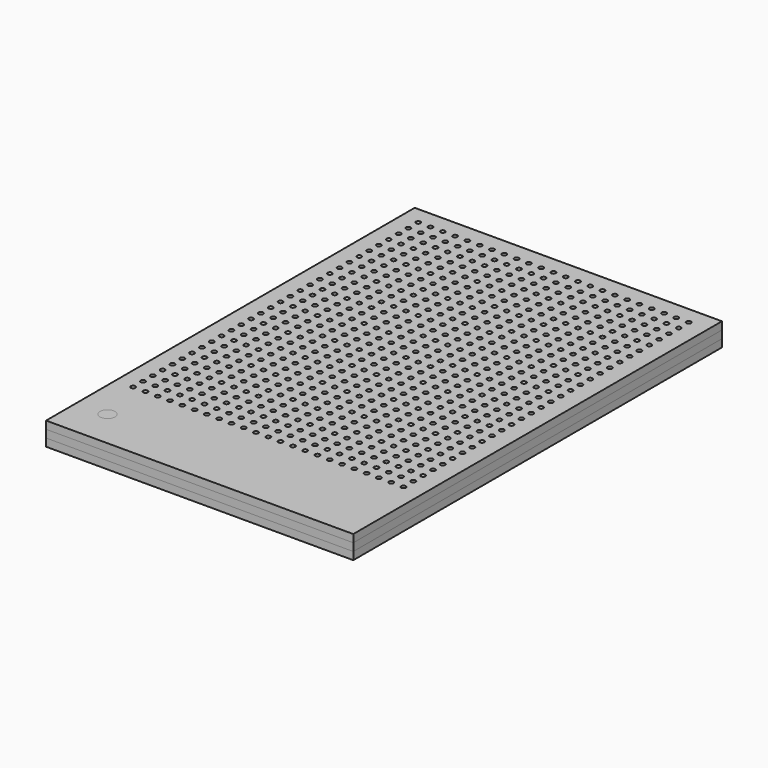
from build123d import *

# Parameters (mm, degrees)
F0_W      = 200
F0_H      = 300
F1_DEPTH  = 5
F2_R      = 1.5
F3_DEPTH  = 5.001
F4_W      = 200
F4_H      = 300
F5_DEPTH  = 5
F6_W      = 3
F6_H      = 235
F7_DEPTH  = 4
F8_R      = 4.875
F9_DEPTH  = 5
F10_DEPTH = 5
F11_R     = 4.875
F12_DEPTH = 0.5


with BuildPart() as f1:
    # F0 (on Top) → F1 (new body)
    with BuildSketch(Plane.XY):
        with Locations((100, 150)):
            Rectangle(F0_W, F0_H)
    extrude(amount=F1_DEPTH)

    # F2 (on face) → F3 (cut, through all)
    with BuildSketch(Plane.XY.offset(5)):
        with Locations((11.5, 288.5)):
            Circle(F2_R)
        with Locations((11.5, 280.5)):
            Circle(F2_R)
        with Locations((11.5, 272.5)):
            Circle(F2_R)
        with Locations((11.5, 264.5)):
            Circle(F2_R)
        with Locations((11.5, 256.5)):
            Circle(F2_R)
        with Locations((11.5, 248.5)):
            Circle(F2_R)
        with Locations((11.5, 240.5)):
            Circle(F2_R)
        with Locations((11.5, 232.5)):
            Circle(F2_R)
        with Locations((11.5, 224.5)):
            Circle(F2_R)
        with Locations((11.5, 216.5)):
            Circle(F2_R)
        with Locations((11.5, 208.5)):
            Circle(F2_R)
        with Locations((11.5, 200.5)):
            Circle(F2_R)
        with Locations((11.5, 192.5)):
            Circle(F2_R)
        with Locations((11.5, 184.5)):
            Circle(F2_R)
        with Locations((11.5, 176.5)):
            Circle(F2_R)
        with Locations((11.5, 168.5)):
            Circle(F2_R)
        with Locations((11.5, 160.5)):
            Circle(F2_R)
        with Locations((11.5, 152.5)):
            Circle(F2_R)
        with Locations((11.5, 144.5)):
            Circle(F2_R)
        with Locations((11.5, 136.5)):
            Circle(F2_R)
        with Locations((11.5, 128.5)):
            Circle(F2_R)
        with Locations((11.5, 120.5)):
            Circle(F2_R)
        with Locations((11.5, 112.5)):
            Circle(F2_R)
        with Locations((11.5, 104.5)):
            Circle(F2_R)
        with Locations((19.5, 288.5)):
            Circle(F2_R)
        with Locations((19.5, 280.5)):
            Circle(F2_R)
        with Locations((19.5, 272.5)):
            Circle(F2_R)
        with Locations((19.5, 264.5)):
            Circle(F2_R)
        with Locations((19.5, 256.5)):
            Circle(F2_R)
        with Locations((19.5, 248.5)):
            Circle(F2_R)
        with Locations((19.5, 240.5)):
            Circle(F2_R)
        with Locations((19.5, 232.5)):
            Circle(F2_R)
        with Locations((19.5, 224.5)):
            Circle(F2_R)
        with Locations((19.5, 216.5)):
            Circle(F2_R)
        with Locations((19.5, 208.5)):
            Circle(F2_R)
        with Locations((19.5, 200.5)):
            Circle(F2_R)
        with Locations((19.5, 192.5)):
            Circle(F2_R)
        with Locations((19.5, 184.5)):
            Circle(F2_R)
        with Locations((19.5, 176.5)):
            Circle(F2_R)
        with Locations((19.5, 168.5)):
            Circle(F2_R)
        with Locations((19.5, 160.5)):
            Circle(F2_R)
        with Locations((19.5, 152.5)):
            Circle(F2_R)
        with Locations((19.5, 144.5)):
            Circle(F2_R)
        with Locations((19.5, 136.5)):
            Circle(F2_R)
        with Locations((19.5, 128.5)):
            Circle(F2_R)
        with Locations((19.5, 120.5)):
            Circle(F2_R)
        with Locations((19.5, 112.5)):
            Circle(F2_R)
        with Locations((19.5, 104.5)):
            Circle(F2_R)
        with Locations((27.5, 288.5)):
            Circle(F2_R)
        with Locations((27.5, 280.5)):
            Circle(F2_R)
        with Locations((27.5, 272.5)):
            Circle(F2_R)
        with Locations((27.5, 264.5)):
            Circle(F2_R)
        with Locations((27.5, 256.5)):
            Circle(F2_R)
        with Locations((27.5, 248.5)):
            Circle(F2_R)
        with Locations((27.5, 240.5)):
            Circle(F2_R)
        with Locations((27.5, 232.5)):
            Circle(F2_R)
        with Locations((27.5, 224.5)):
            Circle(F2_R)
        with Locations((27.5, 216.5)):
            Circle(F2_R)
        with Locations((27.5, 208.5)):
            Circle(F2_R)
        with Locations((27.5, 200.5)):
            Circle(F2_R)
        with Locations((27.5, 192.5)):
            Circle(F2_R)
        with Locations((27.5, 184.5)):
            Circle(F2_R)
        with Locations((27.5, 176.5)):
            Circle(F2_R)
        with Locations((27.5, 168.5)):
            Circle(F2_R)
        with Locations((27.5, 160.5)):
            Circle(F2_R)
        with Locations((27.5, 152.5)):
            Circle(F2_R)
        with Locations((27.5, 144.5)):
            Circle(F2_R)
        with Locations((27.5, 136.5)):
            Circle(F2_R)
        with Locations((27.5, 128.5)):
            Circle(F2_R)
        with Locations((27.5, 120.5)):
            Circle(F2_R)
        with Locations((27.5, 112.5)):
            Circle(F2_R)
        with Locations((27.5, 104.5)):
            Circle(F2_R)
        with Locations((35.5, 288.5)):
            Circle(F2_R)
        with Locations((35.5, 280.5)):
            Circle(F2_R)
        with Locations((35.5, 272.5)):
            Circle(F2_R)
        with Locations((35.5, 264.5)):
            Circle(F2_R)
        with Locations((35.5, 256.5)):
            Circle(F2_R)
        with Locations((35.5, 248.5)):
            Circle(F2_R)
        with Locations((35.5, 240.5)):
            Circle(F2_R)
        with Locations((35.5, 232.5)):
            Circle(F2_R)
        with Locations((35.5, 224.5)):
            Circle(F2_R)
        with Locations((35.5, 216.5)):
            Circle(F2_R)
        with Locations((35.5, 208.5)):
            Circle(F2_R)
        with Locations((35.5, 200.5)):
            Circle(F2_R)
        with Locations((35.5, 192.5)):
            Circle(F2_R)
        with Locations((35.5, 184.5)):
            Circle(F2_R)
        with Locations((35.5, 176.5)):
            Circle(F2_R)
        with Locations((35.5, 168.5)):
            Circle(F2_R)
        with Locations((35.5, 160.5)):
            Circle(F2_R)
        with Locations((35.5, 152.5)):
            Circle(F2_R)
        with Locations((35.5, 144.5)):
            Circle(F2_R)
        with Locations((35.5, 136.5)):
            Circle(F2_R)
        with Locations((35.5, 128.5)):
            Circle(F2_R)
        with Locations((35.5, 120.5)):
            Circle(F2_R)
        with Locations((35.5, 112.5)):
            Circle(F2_R)
        with Locations((35.5, 104.5)):
            Circle(F2_R)
        with Locations((43.5, 288.5)):
            Circle(F2_R)
        with Locations((43.5, 280.5)):
            Circle(F2_R)
        with Locations((43.5, 272.5)):
            Circle(F2_R)
        with Locations((43.5, 264.5)):
            Circle(F2_R)
        with Locations((43.5, 256.5)):
            Circle(F2_R)
        with Locations((43.5, 248.5)):
            Circle(F2_R)
        with Locations((43.5, 240.5)):
            Circle(F2_R)
        with Locations((43.5, 232.5)):
            Circle(F2_R)
        with Locations((43.5, 224.5)):
            Circle(F2_R)
        with Locations((43.5, 216.5)):
            Circle(F2_R)
        with Locations((43.5, 208.5)):
            Circle(F2_R)
        with Locations((43.5, 200.5)):
            Circle(F2_R)
        with Locations((43.5, 192.5)):
            Circle(F2_R)
        with Locations((43.5, 184.5)):
            Circle(F2_R)
        with Locations((43.5, 176.5)):
            Circle(F2_R)
        with Locations((43.5, 168.5)):
            Circle(F2_R)
        with Locations((43.5, 160.5)):
            Circle(F2_R)
        with Locations((43.5, 152.5)):
            Circle(F2_R)
        with Locations((43.5, 144.5)):
            Circle(F2_R)
        with Locations((43.5, 136.5)):
            Circle(F2_R)
        with Locations((43.5, 128.5)):
            Circle(F2_R)
        with Locations((43.5, 120.5)):
            Circle(F2_R)
        with Locations((43.5, 112.5)):
            Circle(F2_R)
        with Locations((43.5, 104.5)):
            Circle(F2_R)
        with Locations((51.5, 288.5)):
            Circle(F2_R)
        with Locations((51.5, 280.5)):
            Circle(F2_R)
        with Locations((51.5, 272.5)):
            Circle(F2_R)
        with Locations((51.5, 264.5)):
            Circle(F2_R)
        with Locations((51.5, 256.5)):
            Circle(F2_R)
        with Locations((51.5, 248.5)):
            Circle(F2_R)
        with Locations((51.5, 240.5)):
            Circle(F2_R)
        with Locations((51.5, 232.5)):
            Circle(F2_R)
        with Locations((51.5, 224.5)):
            Circle(F2_R)
        with Locations((51.5, 216.5)):
            Circle(F2_R)
        with Locations((51.5, 208.5)):
            Circle(F2_R)
        with Locations((51.5, 200.5)):
            Circle(F2_R)
        with Locations((51.5, 192.5)):
            Circle(F2_R)
        with Locations((51.5, 184.5)):
            Circle(F2_R)
        with Locations((51.5, 176.5)):
            Circle(F2_R)
        with Locations((51.5, 168.5)):
            Circle(F2_R)
        with Locations((51.5, 160.5)):
            Circle(F2_R)
        with Locations((51.5, 152.5)):
            Circle(F2_R)
        with Locations((51.5, 144.5)):
            Circle(F2_R)
        with Locations((51.5, 136.5)):
            Circle(F2_R)
        with Locations((51.5, 128.5)):
            Circle(F2_R)
        with Locations((51.5, 120.5)):
            Circle(F2_R)
        with Locations((51.5, 112.5)):
            Circle(F2_R)
        with Locations((51.5, 104.5)):
            Circle(F2_R)
        with Locations((59.5, 288.5)):
            Circle(F2_R)
        with Locations((59.5, 280.5)):
            Circle(F2_R)
        with Locations((59.5, 272.5)):
            Circle(F2_R)
        with Locations((59.5, 264.5)):
            Circle(F2_R)
        with Locations((59.5, 256.5)):
            Circle(F2_R)
        with Locations((59.5, 248.5)):
            Circle(F2_R)
        with Locations((59.5, 240.5)):
            Circle(F2_R)
        with Locations((59.5, 232.5)):
            Circle(F2_R)
        with Locations((59.5, 224.5)):
            Circle(F2_R)
        with Locations((59.5, 216.5)):
            Circle(F2_R)
        with Locations((59.5, 208.5)):
            Circle(F2_R)
        with Locations((59.5, 200.5)):
            Circle(F2_R)
        with Locations((59.5, 192.5)):
            Circle(F2_R)
        with Locations((59.5, 184.5)):
            Circle(F2_R)
        with Locations((59.5, 176.5)):
            Circle(F2_R)
        with Locations((59.5, 168.5)):
            Circle(F2_R)
        with Locations((59.5, 160.5)):
            Circle(F2_R)
        with Locations((59.5, 152.5)):
            Circle(F2_R)
        with Locations((59.5, 144.5)):
            Circle(F2_R)
        with Locations((59.5, 136.5)):
            Circle(F2_R)
        with Locations((59.5, 128.5)):
            Circle(F2_R)
        with Locations((59.5, 120.5)):
            Circle(F2_R)
        with Locations((59.5, 112.5)):
            Circle(F2_R)
        with Locations((59.5, 104.5)):
            Circle(F2_R)
        with Locations((67.5, 288.5)):
            Circle(F2_R)
        with Locations((67.5, 280.5)):
            Circle(F2_R)
        with Locations((67.5, 272.5)):
            Circle(F2_R)
        with Locations((67.5, 264.5)):
            Circle(F2_R)
        with Locations((67.5, 256.5)):
            Circle(F2_R)
        with Locations((67.5, 248.5)):
            Circle(F2_R)
        with Locations((67.5, 240.5)):
            Circle(F2_R)
        with Locations((67.5, 232.5)):
            Circle(F2_R)
        with Locations((67.5, 224.5)):
            Circle(F2_R)
        with Locations((67.5, 216.5)):
            Circle(F2_R)
        with Locations((67.5, 208.5)):
            Circle(F2_R)
        with Locations((67.5, 200.5)):
            Circle(F2_R)
        with Locations((67.5, 192.5)):
            Circle(F2_R)
        with Locations((67.5, 184.5)):
            Circle(F2_R)
        with Locations((67.5, 176.5)):
            Circle(F2_R)
        with Locations((67.5, 168.5)):
            Circle(F2_R)
        with Locations((67.5, 160.5)):
            Circle(F2_R)
        with Locations((67.5, 152.5)):
            Circle(F2_R)
        with Locations((67.5, 144.5)):
            Circle(F2_R)
        with Locations((67.5, 136.5)):
            Circle(F2_R)
        with Locations((67.5, 128.5)):
            Circle(F2_R)
        with Locations((67.5, 120.5)):
            Circle(F2_R)
        with Locations((67.5, 112.5)):
            Circle(F2_R)
        with Locations((67.5, 104.5)):
            Circle(F2_R)
        with Locations((75.5, 288.5)):
            Circle(F2_R)
        with Locations((75.5, 280.5)):
            Circle(F2_R)
        with Locations((75.5, 272.5)):
            Circle(F2_R)
        with Locations((75.5, 264.5)):
            Circle(F2_R)
        with Locations((75.5, 256.5)):
            Circle(F2_R)
        with Locations((75.5, 248.5)):
            Circle(F2_R)
        with Locations((75.5, 240.5)):
            Circle(F2_R)
        with Locations((75.5, 232.5)):
            Circle(F2_R)
        with Locations((75.5, 224.5)):
            Circle(F2_R)
        with Locations((75.5, 216.5)):
            Circle(F2_R)
        with Locations((75.5, 208.5)):
            Circle(F2_R)
        with Locations((75.5, 200.5)):
            Circle(F2_R)
        with Locations((75.5, 192.5)):
            Circle(F2_R)
        with Locations((75.5, 184.5)):
            Circle(F2_R)
        with Locations((75.5, 176.5)):
            Circle(F2_R)
        with Locations((75.5, 168.5)):
            Circle(F2_R)
        with Locations((75.5, 160.5)):
            Circle(F2_R)
        with Locations((75.5, 152.5)):
            Circle(F2_R)
        with Locations((75.5, 144.5)):
            Circle(F2_R)
        with Locations((75.5, 136.5)):
            Circle(F2_R)
        with Locations((75.5, 128.5)):
            Circle(F2_R)
        with Locations((75.5, 120.5)):
            Circle(F2_R)
        with Locations((75.5, 112.5)):
            Circle(F2_R)
        with Locations((75.5, 104.5)):
            Circle(F2_R)
        with Locations((83.5, 288.5)):
            Circle(F2_R)
        with Locations((83.5, 280.5)):
            Circle(F2_R)
        with Locations((83.5, 272.5)):
            Circle(F2_R)
        with Locations((83.5, 264.5)):
            Circle(F2_R)
        with Locations((83.5, 256.5)):
            Circle(F2_R)
        with Locations((83.5, 248.5)):
            Circle(F2_R)
        with Locations((83.5, 240.5)):
            Circle(F2_R)
        with Locations((83.5, 232.5)):
            Circle(F2_R)
        with Locations((83.5, 224.5)):
            Circle(F2_R)
        with Locations((83.5, 216.5)):
            Circle(F2_R)
        with Locations((83.5, 208.5)):
            Circle(F2_R)
        with Locations((83.5, 200.5)):
            Circle(F2_R)
        with Locations((83.5, 192.5)):
            Circle(F2_R)
        with Locations((83.5, 184.5)):
            Circle(F2_R)
        with Locations((83.5, 176.5)):
            Circle(F2_R)
        with Locations((83.5, 168.5)):
            Circle(F2_R)
        with Locations((83.5, 160.5)):
            Circle(F2_R)
        with Locations((83.5, 152.5)):
            Circle(F2_R)
        with Locations((83.5, 144.5)):
            Circle(F2_R)
        with Locations((83.5, 136.5)):
            Circle(F2_R)
        with Locations((83.5, 128.5)):
            Circle(F2_R)
        with Locations((83.5, 120.5)):
            Circle(F2_R)
        with Locations((83.5, 112.5)):
            Circle(F2_R)
        with Locations((83.5, 104.5)):
            Circle(F2_R)
        with Locations((91.5, 288.5)):
            Circle(F2_R)
        with Locations((91.5, 280.5)):
            Circle(F2_R)
        with Locations((91.5, 272.5)):
            Circle(F2_R)
        with Locations((91.5, 264.5)):
            Circle(F2_R)
        with Locations((91.5, 256.5)):
            Circle(F2_R)
        with Locations((91.5, 248.5)):
            Circle(F2_R)
        with Locations((91.5, 240.5)):
            Circle(F2_R)
        with Locations((91.5, 232.5)):
            Circle(F2_R)
        with Locations((91.5, 224.5)):
            Circle(F2_R)
        with Locations((91.5, 216.5)):
            Circle(F2_R)
        with Locations((91.5, 208.5)):
            Circle(F2_R)
        with Locations((91.5, 200.5)):
            Circle(F2_R)
        with Locations((91.5, 192.5)):
            Circle(F2_R)
        with Locations((91.5, 184.5)):
            Circle(F2_R)
        with Locations((91.5, 176.5)):
            Circle(F2_R)
        with Locations((91.5, 168.5)):
            Circle(F2_R)
        with Locations((91.5, 160.5)):
            Circle(F2_R)
        with Locations((91.5, 152.5)):
            Circle(F2_R)
        with Locations((91.5, 144.5)):
            Circle(F2_R)
        with Locations((91.5, 136.5)):
            Circle(F2_R)
        with Locations((91.5, 128.5)):
            Circle(F2_R)
        with Locations((91.5, 120.5)):
            Circle(F2_R)
        with Locations((91.5, 112.5)):
            Circle(F2_R)
        with Locations((91.5, 104.5)):
            Circle(F2_R)
        with Locations((99.5, 288.5)):
            Circle(F2_R)
        with Locations((99.5, 280.5)):
            Circle(F2_R)
        with Locations((99.5, 272.5)):
            Circle(F2_R)
        with Locations((99.5, 264.5)):
            Circle(F2_R)
        with Locations((99.5, 256.5)):
            Circle(F2_R)
        with Locations((99.5, 248.5)):
            Circle(F2_R)
        with Locations((99.5, 240.5)):
            Circle(F2_R)
        with Locations((99.5, 232.5)):
            Circle(F2_R)
        with Locations((99.5, 224.5)):
            Circle(F2_R)
        with Locations((99.5, 216.5)):
            Circle(F2_R)
        with Locations((99.5, 208.5)):
            Circle(F2_R)
        with Locations((99.5, 200.5)):
            Circle(F2_R)
        with Locations((99.5, 192.5)):
            Circle(F2_R)
        with Locations((99.5, 184.5)):
            Circle(F2_R)
        with Locations((99.5, 176.5)):
            Circle(F2_R)
        with Locations((99.5, 168.5)):
            Circle(F2_R)
        with Locations((99.5, 160.5)):
            Circle(F2_R)
        with Locations((99.5, 152.5)):
            Circle(F2_R)
        with Locations((99.5, 144.5)):
            Circle(F2_R)
        with Locations((99.5, 136.5)):
            Circle(F2_R)
        with Locations((99.5, 128.5)):
            Circle(F2_R)
        with Locations((99.5, 120.5)):
            Circle(F2_R)
        with Locations((99.5, 112.5)):
            Circle(F2_R)
        with Locations((99.5, 104.5)):
            Circle(F2_R)
        with Locations((107.5, 288.5)):
            Circle(F2_R)
        with Locations((107.5, 280.5)):
            Circle(F2_R)
        with Locations((107.5, 272.5)):
            Circle(F2_R)
        with Locations((107.5, 264.5)):
            Circle(F2_R)
        with Locations((107.5, 256.5)):
            Circle(F2_R)
        with Locations((107.5, 248.5)):
            Circle(F2_R)
        with Locations((107.5, 240.5)):
            Circle(F2_R)
        with Locations((107.5, 232.5)):
            Circle(F2_R)
        with Locations((107.5, 224.5)):
            Circle(F2_R)
        with Locations((107.5, 216.5)):
            Circle(F2_R)
        with Locations((107.5, 208.5)):
            Circle(F2_R)
        with Locations((107.5, 200.5)):
            Circle(F2_R)
        with Locations((107.5, 192.5)):
            Circle(F2_R)
        with Locations((107.5, 184.5)):
            Circle(F2_R)
        with Locations((107.5, 176.5)):
            Circle(F2_R)
        with Locations((107.5, 168.5)):
            Circle(F2_R)
        with Locations((107.5, 160.5)):
            Circle(F2_R)
        with Locations((107.5, 152.5)):
            Circle(F2_R)
        with Locations((107.5, 144.5)):
            Circle(F2_R)
        with Locations((107.5, 136.5)):
            Circle(F2_R)
        with Locations((107.5, 128.5)):
            Circle(F2_R)
        with Locations((107.5, 120.5)):
            Circle(F2_R)
        with Locations((107.5, 112.5)):
            Circle(F2_R)
        with Locations((107.5, 104.5)):
            Circle(F2_R)
        with Locations((115.5, 288.5)):
            Circle(F2_R)
        with Locations((115.5, 280.5)):
            Circle(F2_R)
        with Locations((115.5, 272.5)):
            Circle(F2_R)
        with Locations((115.5, 264.5)):
            Circle(F2_R)
        with Locations((115.5, 256.5)):
            Circle(F2_R)
        with Locations((115.5, 248.5)):
            Circle(F2_R)
        with Locations((115.5, 240.5)):
            Circle(F2_R)
        with Locations((115.5, 232.5)):
            Circle(F2_R)
        with Locations((115.5, 224.5)):
            Circle(F2_R)
        with Locations((115.5, 216.5)):
            Circle(F2_R)
        with Locations((115.5, 208.5)):
            Circle(F2_R)
        with Locations((115.5, 200.5)):
            Circle(F2_R)
        with Locations((115.5, 192.5)):
            Circle(F2_R)
        with Locations((115.5, 184.5)):
            Circle(F2_R)
        with Locations((115.5, 176.5)):
            Circle(F2_R)
        with Locations((115.5, 168.5)):
            Circle(F2_R)
        with Locations((115.5, 160.5)):
            Circle(F2_R)
        with Locations((115.5, 152.5)):
            Circle(F2_R)
        with Locations((115.5, 144.5)):
            Circle(F2_R)
        with Locations((115.5, 136.5)):
            Circle(F2_R)
        with Locations((115.5, 128.5)):
            Circle(F2_R)
        with Locations((115.5, 120.5)):
            Circle(F2_R)
        with Locations((115.5, 112.5)):
            Circle(F2_R)
        with Locations((115.5, 104.5)):
            Circle(F2_R)
        with Locations((123.5, 288.5)):
            Circle(F2_R)
        with Locations((123.5, 280.5)):
            Circle(F2_R)
        with Locations((123.5, 272.5)):
            Circle(F2_R)
        with Locations((123.5, 264.5)):
            Circle(F2_R)
        with Locations((123.5, 256.5)):
            Circle(F2_R)
        with Locations((123.5, 248.5)):
            Circle(F2_R)
        with Locations((123.5, 240.5)):
            Circle(F2_R)
        with Locations((123.5, 232.5)):
            Circle(F2_R)
        with Locations((123.5, 224.5)):
            Circle(F2_R)
        with Locations((123.5, 216.5)):
            Circle(F2_R)
        with Locations((123.5, 208.5)):
            Circle(F2_R)
        with Locations((123.5, 200.5)):
            Circle(F2_R)
        with Locations((123.5, 192.5)):
            Circle(F2_R)
        with Locations((123.5, 184.5)):
            Circle(F2_R)
        with Locations((123.5, 176.5)):
            Circle(F2_R)
        with Locations((123.5, 168.5)):
            Circle(F2_R)
        with Locations((123.5, 160.5)):
            Circle(F2_R)
        with Locations((123.5, 152.5)):
            Circle(F2_R)
        with Locations((123.5, 144.5)):
            Circle(F2_R)
        with Locations((123.5, 136.5)):
            Circle(F2_R)
        with Locations((123.5, 128.5)):
            Circle(F2_R)
        with Locations((123.5, 120.5)):
            Circle(F2_R)
        with Locations((123.5, 112.5)):
            Circle(F2_R)
        with Locations((123.5, 104.5)):
            Circle(F2_R)
        with Locations((131.5, 288.5)):
            Circle(F2_R)
        with Locations((131.5, 280.5)):
            Circle(F2_R)
        with Locations((131.5, 272.5)):
            Circle(F2_R)
        with Locations((131.5, 264.5)):
            Circle(F2_R)
        with Locations((131.5, 256.5)):
            Circle(F2_R)
        with Locations((131.5, 248.5)):
            Circle(F2_R)
        with Locations((131.5, 240.5)):
            Circle(F2_R)
        with Locations((131.5, 232.5)):
            Circle(F2_R)
        with Locations((131.5, 224.5)):
            Circle(F2_R)
        with Locations((131.5, 216.5)):
            Circle(F2_R)
        with Locations((131.5, 208.5)):
            Circle(F2_R)
        with Locations((131.5, 200.5)):
            Circle(F2_R)
        with Locations((131.5, 192.5)):
            Circle(F2_R)
        with Locations((131.5, 184.5)):
            Circle(F2_R)
        with Locations((131.5, 176.5)):
            Circle(F2_R)
        with Locations((131.5, 168.5)):
            Circle(F2_R)
        with Locations((131.5, 160.5)):
            Circle(F2_R)
        with Locations((131.5, 152.5)):
            Circle(F2_R)
        with Locations((131.5, 144.5)):
            Circle(F2_R)
        with Locations((131.5, 136.5)):
            Circle(F2_R)
        with Locations((131.5, 128.5)):
            Circle(F2_R)
        with Locations((131.5, 120.5)):
            Circle(F2_R)
        with Locations((131.5, 112.5)):
            Circle(F2_R)
        with Locations((131.5, 104.5)):
            Circle(F2_R)
        with Locations((139.5, 288.5)):
            Circle(F2_R)
        with Locations((139.5, 280.5)):
            Circle(F2_R)
        with Locations((139.5, 272.5)):
            Circle(F2_R)
        with Locations((139.5, 264.5)):
            Circle(F2_R)
        with Locations((139.5, 256.5)):
            Circle(F2_R)
        with Locations((139.5, 248.5)):
            Circle(F2_R)
        with Locations((139.5, 240.5)):
            Circle(F2_R)
        with Locations((139.5, 232.5)):
            Circle(F2_R)
        with Locations((139.5, 224.5)):
            Circle(F2_R)
        with Locations((139.5, 216.5)):
            Circle(F2_R)
        with Locations((139.5, 208.5)):
            Circle(F2_R)
        with Locations((139.5, 200.5)):
            Circle(F2_R)
        with Locations((139.5, 192.5)):
            Circle(F2_R)
        with Locations((139.5, 184.5)):
            Circle(F2_R)
        with Locations((139.5, 176.5)):
            Circle(F2_R)
        with Locations((139.5, 168.5)):
            Circle(F2_R)
        with Locations((139.5, 160.5)):
            Circle(F2_R)
        with Locations((139.5, 152.5)):
            Circle(F2_R)
        with Locations((139.5, 144.5)):
            Circle(F2_R)
        with Locations((139.5, 136.5)):
            Circle(F2_R)
        with Locations((139.5, 128.5)):
            Circle(F2_R)
        with Locations((139.5, 120.5)):
            Circle(F2_R)
        with Locations((139.5, 112.5)):
            Circle(F2_R)
        with Locations((139.5, 104.5)):
            Circle(F2_R)
        with Locations((147.5, 288.5)):
            Circle(F2_R)
        with Locations((147.5, 280.5)):
            Circle(F2_R)
        with Locations((147.5, 272.5)):
            Circle(F2_R)
        with Locations((147.5, 264.5)):
            Circle(F2_R)
        with Locations((147.5, 256.5)):
            Circle(F2_R)
        with Locations((147.5, 248.5)):
            Circle(F2_R)
        with Locations((147.5, 240.5)):
            Circle(F2_R)
        with Locations((147.5, 232.5)):
            Circle(F2_R)
        with Locations((147.5, 224.5)):
            Circle(F2_R)
        with Locations((147.5, 216.5)):
            Circle(F2_R)
        with Locations((147.5, 208.5)):
            Circle(F2_R)
        with Locations((147.5, 200.5)):
            Circle(F2_R)
        with Locations((147.5, 192.5)):
            Circle(F2_R)
        with Locations((147.5, 184.5)):
            Circle(F2_R)
        with Locations((147.5, 176.5)):
            Circle(F2_R)
        with Locations((147.5, 168.5)):
            Circle(F2_R)
        with Locations((147.5, 160.5)):
            Circle(F2_R)
        with Locations((147.5, 152.5)):
            Circle(F2_R)
        with Locations((147.5, 144.5)):
            Circle(F2_R)
        with Locations((147.5, 136.5)):
            Circle(F2_R)
        with Locations((147.5, 128.5)):
            Circle(F2_R)
        with Locations((147.5, 120.5)):
            Circle(F2_R)
        with Locations((147.5, 112.5)):
            Circle(F2_R)
        with Locations((147.5, 104.5)):
            Circle(F2_R)
        with Locations((155.5, 288.5)):
            Circle(F2_R)
        with Locations((155.5, 280.5)):
            Circle(F2_R)
        with Locations((155.5, 272.5)):
            Circle(F2_R)
        with Locations((155.5, 264.5)):
            Circle(F2_R)
        with Locations((155.5, 256.5)):
            Circle(F2_R)
        with Locations((155.5, 248.5)):
            Circle(F2_R)
        with Locations((155.5, 240.5)):
            Circle(F2_R)
        with Locations((155.5, 232.5)):
            Circle(F2_R)
        with Locations((155.5, 224.5)):
            Circle(F2_R)
        with Locations((155.5, 216.5)):
            Circle(F2_R)
        with Locations((155.5, 208.5)):
            Circle(F2_R)
        with Locations((155.5, 200.5)):
            Circle(F2_R)
        with Locations((155.5, 192.5)):
            Circle(F2_R)
        with Locations((155.5, 184.5)):
            Circle(F2_R)
        with Locations((155.5, 176.5)):
            Circle(F2_R)
        with Locations((155.5, 168.5)):
            Circle(F2_R)
        with Locations((155.5, 160.5)):
            Circle(F2_R)
        with Locations((155.5, 152.5)):
            Circle(F2_R)
        with Locations((155.5, 144.5)):
            Circle(F2_R)
        with Locations((155.5, 136.5)):
            Circle(F2_R)
        with Locations((155.5, 128.5)):
            Circle(F2_R)
        with Locations((155.5, 120.5)):
            Circle(F2_R)
        with Locations((155.5, 112.5)):
            Circle(F2_R)
        with Locations((155.5, 104.5)):
            Circle(F2_R)
        with Locations((163.5, 288.5)):
            Circle(F2_R)
        with Locations((163.5, 280.5)):
            Circle(F2_R)
        with Locations((163.5, 272.5)):
            Circle(F2_R)
        with Locations((163.5, 264.5)):
            Circle(F2_R)
        with Locations((163.5, 256.5)):
            Circle(F2_R)
        with Locations((163.5, 248.5)):
            Circle(F2_R)
        with Locations((163.5, 240.5)):
            Circle(F2_R)
        with Locations((163.5, 232.5)):
            Circle(F2_R)
        with Locations((163.5, 224.5)):
            Circle(F2_R)
        with Locations((163.5, 216.5)):
            Circle(F2_R)
        with Locations((163.5, 208.5)):
            Circle(F2_R)
        with Locations((163.5, 200.5)):
            Circle(F2_R)
        with Locations((163.5, 192.5)):
            Circle(F2_R)
        with Locations((163.5, 184.5)):
            Circle(F2_R)
        with Locations((163.5, 176.5)):
            Circle(F2_R)
        with Locations((163.5, 168.5)):
            Circle(F2_R)
        with Locations((163.5, 160.5)):
            Circle(F2_R)
        with Locations((163.5, 152.5)):
            Circle(F2_R)
        with Locations((163.5, 144.5)):
            Circle(F2_R)
        with Locations((163.5, 136.5)):
            Circle(F2_R)
        with Locations((163.5, 128.5)):
            Circle(F2_R)
        with Locations((163.5, 120.5)):
            Circle(F2_R)
        with Locations((163.5, 112.5)):
            Circle(F2_R)
        with Locations((163.5, 104.5)):
            Circle(F2_R)
        with Locations((171.5, 288.5)):
            Circle(F2_R)
        with Locations((171.5, 280.5)):
            Circle(F2_R)
        with Locations((171.5, 272.5)):
            Circle(F2_R)
        with Locations((171.5, 264.5)):
            Circle(F2_R)
        with Locations((171.5, 256.5)):
            Circle(F2_R)
        with Locations((171.5, 248.5)):
            Circle(F2_R)
        with Locations((171.5, 240.5)):
            Circle(F2_R)
        with Locations((171.5, 232.5)):
            Circle(F2_R)
        with Locations((171.5, 224.5)):
            Circle(F2_R)
        with Locations((171.5, 216.5)):
            Circle(F2_R)
        with Locations((171.5, 208.5)):
            Circle(F2_R)
        with Locations((171.5, 200.5)):
            Circle(F2_R)
        with Locations((171.5, 192.5)):
            Circle(F2_R)
        with Locations((171.5, 184.5)):
            Circle(F2_R)
        with Locations((171.5, 176.5)):
            Circle(F2_R)
        with Locations((171.5, 168.5)):
            Circle(F2_R)
        with Locations((171.5, 160.5)):
            Circle(F2_R)
        with Locations((171.5, 152.5)):
            Circle(F2_R)
        with Locations((171.5, 144.5)):
            Circle(F2_R)
        with Locations((171.5, 136.5)):
            Circle(F2_R)
        with Locations((171.5, 128.5)):
            Circle(F2_R)
        with Locations((171.5, 120.5)):
            Circle(F2_R)
        with Locations((171.5, 112.5)):
            Circle(F2_R)
        with Locations((171.5, 104.5)):
            Circle(F2_R)
        with Locations((179.5, 288.5)):
            Circle(F2_R)
        with Locations((179.5, 280.5)):
            Circle(F2_R)
        with Locations((179.5, 272.5)):
            Circle(F2_R)
        with Locations((179.5, 264.5)):
            Circle(F2_R)
        with Locations((179.5, 256.5)):
            Circle(F2_R)
        with Locations((179.5, 248.5)):
            Circle(F2_R)
        with Locations((179.5, 240.5)):
            Circle(F2_R)
        with Locations((179.5, 232.5)):
            Circle(F2_R)
        with Locations((179.5, 224.5)):
            Circle(F2_R)
        with Locations((179.5, 216.5)):
            Circle(F2_R)
        with Locations((179.5, 208.5)):
            Circle(F2_R)
        with Locations((179.5, 200.5)):
            Circle(F2_R)
        with Locations((179.5, 192.5)):
            Circle(F2_R)
        with Locations((179.5, 184.5)):
            Circle(F2_R)
        with Locations((179.5, 176.5)):
            Circle(F2_R)
        with Locations((179.5, 168.5)):
            Circle(F2_R)
        with Locations((179.5, 160.5)):
            Circle(F2_R)
        with Locations((179.5, 152.5)):
            Circle(F2_R)
        with Locations((179.5, 144.5)):
            Circle(F2_R)
        with Locations((179.5, 136.5)):
            Circle(F2_R)
        with Locations((179.5, 128.5)):
            Circle(F2_R)
        with Locations((179.5, 120.5)):
            Circle(F2_R)
        with Locations((179.5, 112.5)):
            Circle(F2_R)
        with Locations((179.5, 104.5)):
            Circle(F2_R)
        with Locations((187.5, 288.5)):
            Circle(F2_R)
        with Locations((187.5, 280.5)):
            Circle(F2_R)
        with Locations((187.5, 272.5)):
            Circle(F2_R)
        with Locations((187.5, 264.5)):
            Circle(F2_R)
        with Locations((187.5, 256.5)):
            Circle(F2_R)
        with Locations((187.5, 248.5)):
            Circle(F2_R)
        with Locations((187.5, 240.5)):
            Circle(F2_R)
        with Locations((187.5, 232.5)):
            Circle(F2_R)
        with Locations((187.5, 224.5)):
            Circle(F2_R)
        with Locations((187.5, 216.5)):
            Circle(F2_R)
        with Locations((187.5, 208.5)):
            Circle(F2_R)
        with Locations((187.5, 200.5)):
            Circle(F2_R)
        with Locations((187.5, 192.5)):
            Circle(F2_R)
        with Locations((187.5, 184.5)):
            Circle(F2_R)
        with Locations((187.5, 176.5)):
            Circle(F2_R)
        with Locations((187.5, 168.5)):
            Circle(F2_R)
        with Locations((187.5, 160.5)):
            Circle(F2_R)
        with Locations((187.5, 152.5)):
            Circle(F2_R)
        with Locations((187.5, 144.5)):
            Circle(F2_R)
        with Locations((187.5, 136.5)):
            Circle(F2_R)
        with Locations((187.5, 128.5)):
            Circle(F2_R)
        with Locations((187.5, 120.5)):
            Circle(F2_R)
        with Locations((187.5, 112.5)):
            Circle(F2_R)
        with Locations((187.5, 104.5)):
            Circle(F2_R)
        with Locations((11.5, 96.5)):
            Circle(F2_R)
        with Locations((11.5, 88.5)):
            Circle(F2_R)
        with Locations((11.5, 80.5)):
            Circle(F2_R)
        with Locations((11.5, 72.5)):
            Circle(F2_R)
        with Locations((11.5, 64.5)):
            Circle(F2_R)
        with Locations((11.5, 56.5)):
            Circle(F2_R)
        with Locations((19.5, 96.5)):
            Circle(F2_R)
        with Locations((19.5, 88.5)):
            Circle(F2_R)
        with Locations((19.5, 80.5)):
            Circle(F2_R)
        with Locations((19.5, 72.5)):
            Circle(F2_R)
        with Locations((19.5, 64.5)):
            Circle(F2_R)
        with Locations((19.5, 56.5)):
            Circle(F2_R)
        with Locations((27.5, 96.5)):
            Circle(F2_R)
        with Locations((27.5, 88.5)):
            Circle(F2_R)
        with Locations((27.5, 80.5)):
            Circle(F2_R)
        with Locations((27.5, 72.5)):
            Circle(F2_R)
        with Locations((27.5, 64.5)):
            Circle(F2_R)
        with Locations((27.5, 56.5)):
            Circle(F2_R)
        with Locations((35.5, 96.5)):
            Circle(F2_R)
        with Locations((35.5, 88.5)):
            Circle(F2_R)
        with Locations((35.5, 80.5)):
            Circle(F2_R)
        with Locations((35.5, 72.5)):
            Circle(F2_R)
        with Locations((35.5, 64.5)):
            Circle(F2_R)
        with Locations((35.5, 56.5)):
            Circle(F2_R)
        with Locations((43.5, 96.5)):
            Circle(F2_R)
        with Locations((43.5, 88.5)):
            Circle(F2_R)
        with Locations((43.5, 80.5)):
            Circle(F2_R)
        with Locations((43.5, 72.5)):
            Circle(F2_R)
        with Locations((43.5, 64.5)):
            Circle(F2_R)
        with Locations((43.5, 56.5)):
            Circle(F2_R)
        with Locations((51.5, 96.5)):
            Circle(F2_R)
        with Locations((51.5, 88.5)):
            Circle(F2_R)
        with Locations((51.5, 80.5)):
            Circle(F2_R)
        with Locations((51.5, 72.5)):
            Circle(F2_R)
        with Locations((51.5, 64.5)):
            Circle(F2_R)
        with Locations((51.5, 56.5)):
            Circle(F2_R)
        with Locations((59.5, 96.5)):
            Circle(F2_R)
        with Locations((59.5, 88.5)):
            Circle(F2_R)
        with Locations((59.5, 80.5)):
            Circle(F2_R)
        with Locations((59.5, 72.5)):
            Circle(F2_R)
        with Locations((59.5, 64.5)):
            Circle(F2_R)
        with Locations((59.5, 56.5)):
            Circle(F2_R)
        with Locations((67.5, 96.5)):
            Circle(F2_R)
        with Locations((67.5, 88.5)):
            Circle(F2_R)
        with Locations((67.5, 80.5)):
            Circle(F2_R)
        with Locations((67.5, 72.5)):
            Circle(F2_R)
        with Locations((67.5, 64.5)):
            Circle(F2_R)
        with Locations((67.5, 56.5)):
            Circle(F2_R)
        with Locations((75.5, 96.5)):
            Circle(F2_R)
        with Locations((75.5, 88.5)):
            Circle(F2_R)
        with Locations((75.5, 80.5)):
            Circle(F2_R)
        with Locations((75.5, 72.5)):
            Circle(F2_R)
        with Locations((75.5, 64.5)):
            Circle(F2_R)
        with Locations((75.5, 56.5)):
            Circle(F2_R)
        with Locations((83.5, 96.5)):
            Circle(F2_R)
        with Locations((83.5, 88.5)):
            Circle(F2_R)
        with Locations((83.5, 80.5)):
            Circle(F2_R)
        with Locations((83.5, 72.5)):
            Circle(F2_R)
        with Locations((83.5, 64.5)):
            Circle(F2_R)
        with Locations((83.5, 56.5)):
            Circle(F2_R)
        with Locations((91.5, 96.5)):
            Circle(F2_R)
        with Locations((91.5, 88.5)):
            Circle(F2_R)
        with Locations((91.5, 80.5)):
            Circle(F2_R)
        with Locations((91.5, 72.5)):
            Circle(F2_R)
        with Locations((91.5, 64.5)):
            Circle(F2_R)
        with Locations((91.5, 56.5)):
            Circle(F2_R)
        with Locations((99.5, 96.5)):
            Circle(F2_R)
        with Locations((99.5, 88.5)):
            Circle(F2_R)
        with Locations((99.5, 80.5)):
            Circle(F2_R)
        with Locations((99.5, 72.5)):
            Circle(F2_R)
        with Locations((99.5, 64.5)):
            Circle(F2_R)
        with Locations((99.5, 56.5)):
            Circle(F2_R)
        with Locations((107.5, 96.5)):
            Circle(F2_R)
        with Locations((107.5, 88.5)):
            Circle(F2_R)
        with Locations((107.5, 80.5)):
            Circle(F2_R)
        with Locations((107.5, 72.5)):
            Circle(F2_R)
        with Locations((107.5, 64.5)):
            Circle(F2_R)
        with Locations((107.5, 56.5)):
            Circle(F2_R)
        with Locations((115.5, 96.5)):
            Circle(F2_R)
        with Locations((115.5, 88.5)):
            Circle(F2_R)
        with Locations((115.5, 80.5)):
            Circle(F2_R)
        with Locations((115.5, 72.5)):
            Circle(F2_R)
        with Locations((115.5, 64.5)):
            Circle(F2_R)
        with Locations((115.5, 56.5)):
            Circle(F2_R)
        with Locations((123.5, 96.5)):
            Circle(F2_R)
        with Locations((123.5, 88.5)):
            Circle(F2_R)
        with Locations((123.5, 80.5)):
            Circle(F2_R)
        with Locations((123.5, 72.5)):
            Circle(F2_R)
        with Locations((123.5, 64.5)):
            Circle(F2_R)
        with Locations((123.5, 56.5)):
            Circle(F2_R)
        with Locations((131.5, 96.5)):
            Circle(F2_R)
        with Locations((131.5, 88.5)):
            Circle(F2_R)
        with Locations((131.5, 80.5)):
            Circle(F2_R)
        with Locations((131.5, 72.5)):
            Circle(F2_R)
        with Locations((131.5, 64.5)):
            Circle(F2_R)
        with Locations((131.5, 56.5)):
            Circle(F2_R)
        with Locations((139.5, 96.5)):
            Circle(F2_R)
        with Locations((139.5, 88.5)):
            Circle(F2_R)
        with Locations((139.5, 80.5)):
            Circle(F2_R)
        with Locations((139.5, 72.5)):
            Circle(F2_R)
        with Locations((139.5, 64.5)):
            Circle(F2_R)
        with Locations((139.5, 56.5)):
            Circle(F2_R)
        with Locations((147.5, 96.5)):
            Circle(F2_R)
        with Locations((147.5, 88.5)):
            Circle(F2_R)
        with Locations((147.5, 80.5)):
            Circle(F2_R)
        with Locations((147.5, 72.5)):
            Circle(F2_R)
        with Locations((147.5, 64.5)):
            Circle(F2_R)
        with Locations((147.5, 56.5)):
            Circle(F2_R)
        with Locations((155.5, 96.5)):
            Circle(F2_R)
        with Locations((155.5, 88.5)):
            Circle(F2_R)
        with Locations((155.5, 80.5)):
            Circle(F2_R)
        with Locations((155.5, 72.5)):
            Circle(F2_R)
        with Locations((155.5, 64.5)):
            Circle(F2_R)
        with Locations((155.5, 56.5)):
            Circle(F2_R)
        with Locations((163.5, 96.5)):
            Circle(F2_R)
        with Locations((163.5, 88.5)):
            Circle(F2_R)
        with Locations((163.5, 80.5)):
            Circle(F2_R)
        with Locations((163.5, 72.5)):
            Circle(F2_R)
        with Locations((163.5, 64.5)):
            Circle(F2_R)
        with Locations((163.5, 56.5)):
            Circle(F2_R)
        with Locations((171.5, 96.5)):
            Circle(F2_R)
        with Locations((171.5, 88.5)):
            Circle(F2_R)
        with Locations((171.5, 80.5)):
            Circle(F2_R)
        with Locations((171.5, 72.5)):
            Circle(F2_R)
        with Locations((171.5, 64.5)):
            Circle(F2_R)
        with Locations((171.5, 56.5)):
            Circle(F2_R)
        with Locations((179.5, 96.5)):
            Circle(F2_R)
        with Locations((179.5, 88.5)):
            Circle(F2_R)
        with Locations((179.5, 80.5)):
            Circle(F2_R)
        with Locations((179.5, 72.5)):
            Circle(F2_R)
        with Locations((179.5, 64.5)):
            Circle(F2_R)
        with Locations((179.5, 56.5)):
            Circle(F2_R)
        with Locations((187.5, 96.5)):
            Circle(F2_R)
        with Locations((187.5, 88.5)):
            Circle(F2_R)
        with Locations((187.5, 80.5)):
            Circle(F2_R)
        with Locations((187.5, 72.5)):
            Circle(F2_R)
        with Locations((187.5, 64.5)):
            Circle(F2_R)
        with Locations((187.5, 56.5)):
            Circle(F2_R)
    extrude(amount=-F3_DEPTH, mode=Mode.SUBTRACT)

    # F8 (on face) → F9 (cut)
    with BuildSketch(Plane.XY.offset(5)):
        with Locations((20, 25)):
            Circle(F8_R)
    extrude(amount=-F9_DEPTH, mode=Mode.SUBTRACT)


with BuildPart() as f5:
    # F4 (on face) → F5 (new body)
    with BuildSketch(Plane(origin=(0, 0, 0), x_dir=(1, 0, 0), z_dir=(0, 0, -1))):
        with Locations((100, -150)):
            Rectangle(F4_W, F4_H)
    extrude(amount=F5_DEPTH)

    # F6 (on face) → F7 (cut)
    with BuildSketch(Plane.XY):
        with Locations((11.5, 172.5)):
            Rectangle(F6_W, F6_H)
        with BuildLine():
            Line((13, 55), (10, 55))
            Line((10, 55), (10, 25))
            ThreePointArc((10, 25), (12.9289321881, 17.9289321881), (20, 15))
            Line((20, 15), (179, 15))
            ThreePointArc((179, 15), (186.0710678119, 17.9289321881), (189, 25))
            Line((189, 25), (189, 55))
            Line((189, 55), (186, 55))
            Line((186, 55), (181, 55))
            Line((181, 55), (178, 55))
            Line((178, 55), (173, 55))
            Line((173, 55), (170, 55))
            Line((170, 55), (165, 55))
            Line((165, 55), (162, 55))
            Line((162, 55), (157, 55))
            Line((157, 55), (154, 55))
            Line((154, 55), (149, 55))
            Line((149, 55), (146, 55))
            Line((146, 55), (141, 55))
            Line((141, 55), (138, 55))
            Line((138, 55), (133, 55))
            Line((133, 55), (130, 55))
            Line((130, 55), (125, 55))
            Line((125, 55), (122, 55))
            Line((122, 55), (117, 55))
            Line((117, 55), (114, 55))
            Line((114, 55), (109, 55))
            Line((109, 55), (106, 55))
            Line((106, 55), (101, 55))
            Line((101, 55), (98, 55))
            Line((98, 55), (93, 55))
            Line((93, 55), (90, 55))
            Line((90, 55), (85, 55))
            Line((85, 55), (82, 55))
            Line((82, 55), (77, 55))
            Line((77, 55), (74, 55))
            Line((74, 55), (69, 55))
            Line((69, 55), (66, 55))
            Line((66, 55), (61, 55))
            Line((61, 55), (58, 55))
            Line((58, 55), (53, 55))
            Line((53, 55), (50, 55))
            Line((50, 55), (45, 55))
            Line((45, 55), (42, 55))
            Line((42, 55), (37, 55))
            Line((37, 55), (34, 55))
            Line((34, 55), (29, 55))
            Line((29, 55), (26, 55))
            Line((26, 55), (21, 55))
            Line((21, 55), (18, 55))
            Line((18, 55), (13, 55))
        make_face()
        with Locations((19.5, 172.5)):
            Rectangle(F6_W, F6_H)
        with Locations((27.5, 172.5)):
            Rectangle(F6_W, F6_H)
        with Locations((187.5, 172.5)):
            Rectangle(F6_W, F6_H)
        with Locations((35.5, 172.5)):
            Rectangle(F6_W, F6_H)
        with Locations((179.5, 172.5)):
            Rectangle(F6_W, F6_H)
        with Locations((43.5, 172.5)):
            Rectangle(F6_W, F6_H)
        with Locations((171.5, 172.5)):
            Rectangle(F6_W, F6_H)
        with Locations((51.5, 172.5)):
            Rectangle(F6_W, F6_H)
        with Locations((163.5, 172.5)):
            Rectangle(F6_W, F6_H)
        with Locations((59.5, 172.5)):
            Rectangle(F6_W, F6_H)
        with Locations((155.5, 172.5)):
            Rectangle(F6_W, F6_H)
        with Locations((67.5, 172.5)):
            Rectangle(F6_W, F6_H)
        with Locations((147.5, 172.5)):
            Rectangle(F6_W, F6_H)
        with Locations((75.5, 172.5)):
            Rectangle(F6_W, F6_H)
        with Locations((139.5, 172.5)):
            Rectangle(F6_W, F6_H)
        with Locations((83.5, 172.5)):
            Rectangle(F6_W, F6_H)
        with Locations((131.5, 172.5)):
            Rectangle(F6_W, F6_H)
        with Locations((91.5, 172.5)):
            Rectangle(F6_W, F6_H)
        with Locations((123.5, 172.5)):
            Rectangle(F6_W, F6_H)
        with Locations((99.5, 172.5)):
            Rectangle(F6_W, F6_H)
        with Locations((115.5, 172.5)):
            Rectangle(F6_W, F6_H)
        with Locations((107.5, 172.5)):
            Rectangle(F6_W, F6_H)
    extrude(amount=-F7_DEPTH, mode=Mode.SUBTRACT)


with BuildPart() as f10:
    # F10 (new): a face of the model
    f10_faces = [f5.part.faces().sort_by_distance(p)[0] for p in [
        (100, 150, -5),
    ]]
    extrude(f10_faces, amount=F10_DEPTH)


with BuildPart() as f12:
    # F11 (on face) → F12 (new body)
    with BuildSketch(Plane.XY.offset(5)):
        with Locations((20, 25)):
            Circle(F11_R)
    extrude(amount=-F12_DEPTH)


solid = Compound([f1.part, f5.part, f10.part, f12.part])
